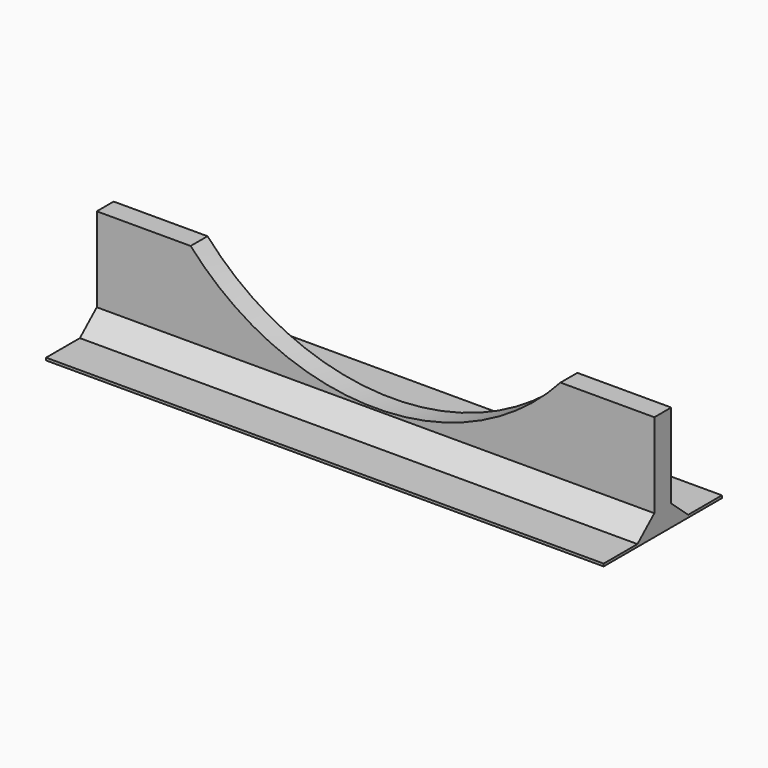
from build123d import *

# Parameters (mm, degrees)
F1_DEPTH = 3.175
F3_DEPTH = 167.64


# Not quite as in the source:
# - a pattern or mirror of a feature is missing from the dataset's text; its kind, count and spacing are read off the source's solid


with BuildPart() as f1:
    # F0 (on Front) → F1 (new body, symmetric)
    with BuildSketch(Plane.XZ):
        with BuildLine():
            ThreePointArc((55.5949879174, -49.7616566718), (0, -74.6125), (-55.5949879174, -49.7616566718))
            Line((-55.5949879174, -49.7616566718), (-83.82, -49.7616566718))
            Line((-83.82, -49.7616566718), (-83.82, -81.5116566718))
            Line((-83.82, -81.5116566718), (83.82, -81.5116566718))
            Line((83.82, -81.5116566718), (83.82, -49.7616566718))
            Line((83.82, -49.7616566718), (55.5949879174, -49.7616566718))
        make_face()
    extrude(amount=F1_DEPTH, both=True)

    # F2 (on face) → F3 (join, through all)
    with BuildSketch(Plane.YZ.offset(83.82)):
        Polygon((-3.175, -81.5116566718), (-3.175, -75.1616566718), (-9.525, -80.7496566718), (-22.225, -80.7496566718), (-22.225, -81.5116566718), (-10.3909090909, -81.5116566718), align=None)
    f3 = extrude(amount=-F3_DEPTH)

    # F3_copies: F3 across plane
    add(f3.mirror(Plane.ZX))


solid = f1.part
